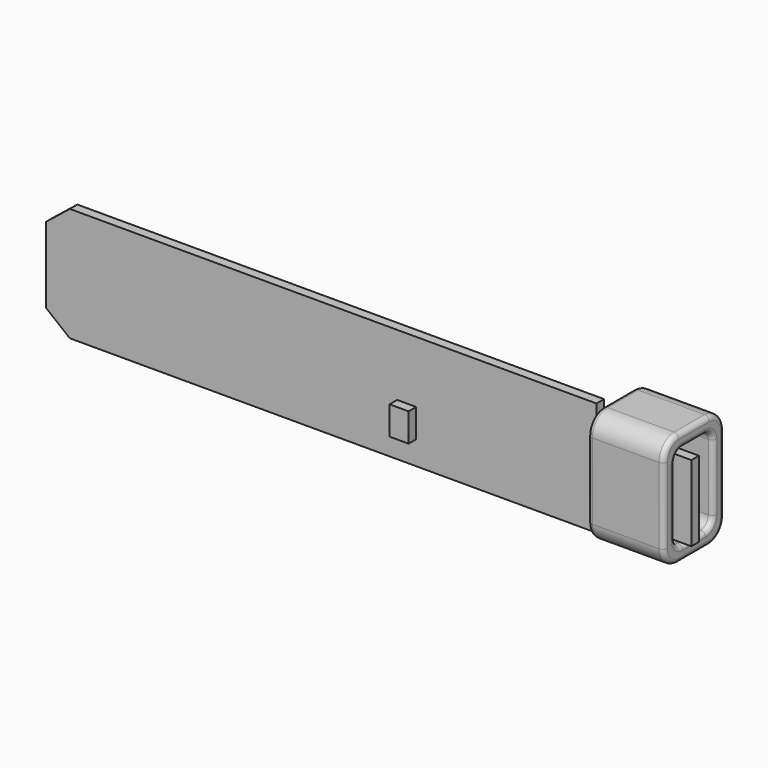
from build123d import *

# Parameters (mm, degrees)
F1_DEPTH  = 1
F4_DEPTH  = 8
F5_R      = 0.5
F6_W      = 2
F6_H      = 0.5
F7_DEPTH  = 0.5
F8_R      = 0.24999
F9_W      = 2
F9_H      = 3
F10_DEPTH = 2


# Not quite as in the source:
# - a fillet or chamfer is up to 0.001 mm smaller than in the source, because OpenCascade refuses the exact size


with BuildPart() as f1:
    # F0 (on Front) → F1 (new body)
    with BuildSketch(Plane.XZ):
        with BuildLine():
            Line((-42.178902775, 4), (-42.178902775, 0))
            Line((-42.178902775, 0), (-42.178902775, -4))
            Line((-42.178902775, -4), (-39.678902775, -6))
            Line((-39.678902775, -6), (15.821097225, -6))
            Line((15.821097225, -6), (15.821097225, -4.5))
            ThreePointArc((15.821097225, -4.5), (15.9675438344, -4.1464466094), (16.321097225, -4))
            Line((16.321097225, -4), (25.821097225, -4))
            Line((25.821097225, -4), (25.821097225, 0))
            Line((25.821097225, 0), (25.821097225, 4))
            Line((25.821097225, 4), (16.321097225, 4))
            ThreePointArc((16.321097225, 4), (15.9675438344, 4.1464466094), (15.821097225, 4.5))
            Line((15.821097225, 4.5), (15.821097225, 6))
            Line((15.821097225, 6), (-39.678902775, 6))
            Line((-39.678902775, 6), (-42.178902775, 4))
        make_face()
    extrude(amount=F1_DEPTH)



with BuildPart() as f4:
    # F3 (on offset) → F4 (new body)
    with BuildSketch(Plane.YZ.offset(16.5)):
        with BuildLine():
            Line((-1, -6), (3, -6))
            ThreePointArc((3, -6), (4.4142135624, -5.4142135624), (5, -4))
            Line((5, -4), (5, 4))
            ThreePointArc((5, 4), (4.4142135624, 5.4142135624), (3, 6))
            Line((3, 6), (-1, 6))
            ThreePointArc((-1, 6), (-2.4142135624, 5.4142135624), (-3, 4))
            Line((-3, 4), (-3, -4))
            ThreePointArc((-3, -4), (-2.4142135624, -5.4142135624), (-1, -6))
        make_face()
        with BuildLine():
            ThreePointArc((3.5, -3.5), (3.2071067812, -4.2071067812), (2.5, -4.5))
            Line((2.5, -4.5), (-0.5, -4.5))
            ThreePointArc((-0.5, -4.5), (-1.2071067812, -4.2071067812), (-1.5, -3.5))
            Line((-1.5, -3.5), (-1.5, 3.5))
            ThreePointArc((-1.5, 3.5), (-1.2071067812, 4.2071067812), (-0.5, 4.5))
            Line((-0.5, 4.5), (2.5, 4.5))
            ThreePointArc((2.5, 4.5), (3.2071067812, 4.2071067812), (3.5, 3.5))
            Line((3.5, 3.5), (3.5, -3.5))
        make_face(mode=Mode.SUBTRACT)
    extrude(amount=F4_DEPTH)

    # F5
    f5_edges = [f4.edges().sort_by_distance(p)[0] for p in [
        (24.5, -2.414214, 5.414214),
        (24.5, -1.207107, 4.207107),
        (16.5, -1.207107, 4.207107),
        (16.5, -2.414214, 5.414214),
    ]]
    fillet(f5_edges, radius=F5_R)


with BuildPart() as f1_1:
    add(f1.part)

    add(f4.part)  # F7 merges F4
    # F6 (on offset) → F7 (join)
    with BuildSketch(Plane.YZ.offset(16.5)):
        with Locations((-1.159823034, 0)):
            Rectangle(F6_W, F6_H)
    extrude(amount=F7_DEPTH)

    # F8 (radius 0.25 in the source; OpenCascade refuses exactly that, so slightly less here)
    f8_edges = [f1_1.edges().sort_by_distance(p)[0] for p in [
        (17, -1.25, 0.25),
        (17, -1.25, -0.25),
        (16.5, -1.5, -0.25),
        (16.5, -1.5, 0.25),
    ]]
    fillet(f8_edges, radius=F8_R)

    # F9 (on Front) → F10 (join)
    with BuildSketch(Plane.XZ):
        with Locations((-4.178902775, -2)):
            Rectangle(F9_W, F9_H)
    extrude(amount=F10_DEPTH)


solid = f1_1.part
